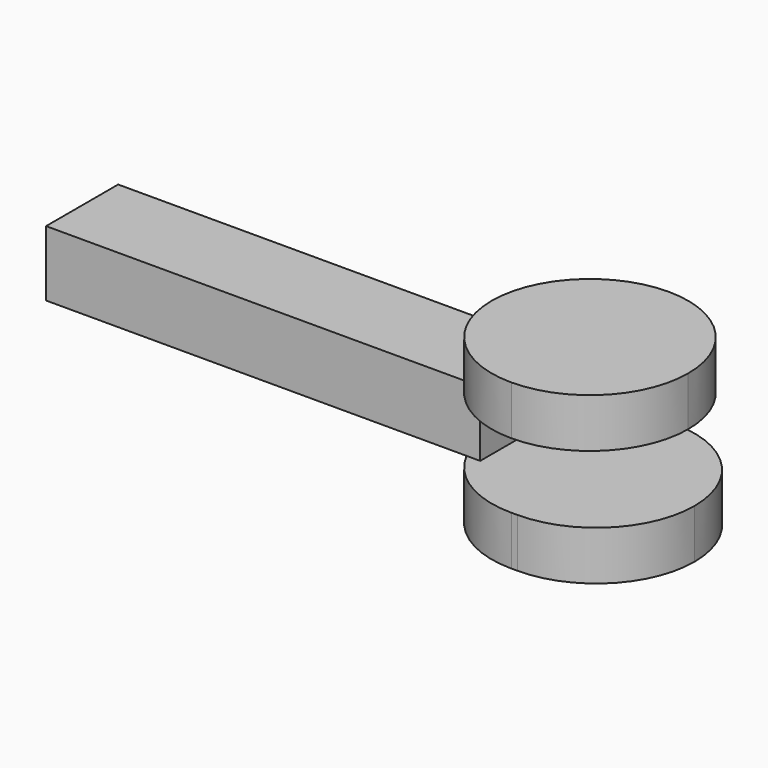
from build123d import *

# Parameters (mm, degrees)
F1_DEPTH = 24
F2_DEPTH = 11
F3_R     = 23.99999
F3_2_R   = 23.99999


# Not quite as in the source:
# - a fillet or chamfer is up to 0.001 mm smaller than in the source, because OpenCascade refuses the exact size


with BuildPart() as f1:
    # F0 (on Front) → F1 (new body, symmetric)
    with BuildSketch(Plane.XZ):
        Polygon((28.0138015747, 20.5115029328), (28.0138015747, 8.5115029328), (34.0138015747, 8.5115029328), (76.0138015747, 8.5115029328), (76.0138015747, 20.5115029328), align=None)
    extrude(amount=F1_DEPTH, both=True)

    # F3 (radius 24 in the source; OpenCascade refuses exactly that, so slightly less here)
    f3_edges = [f1.edges().sort_by_distance(p)[0] for p in [
        (76.013802, -24, 14.511503),
        (76.013802, 24, 14.511503),
        (28.013802, -24, 14.511503),
        (28.013802, 24, 14.511503),
    ]]
    fillet(f3_edges, radius=F3_R)


with BuildPart() as f1b:
    # F0 (on Front) → F1, piece 2 (new body, symmetric)
    with BuildSketch(Plane.XZ):
        Polygon((34.0138015747, -7.4884970672), (28.0138015747, -7.4884970672), (28.0138015747, -19.4884970672), (77.5421783328, -19.4884970672), (77.5421783328, -7.4884970672), align=None)
    extrude(amount=F1_DEPTH, both=True)

    # F3#2 (radius 24 in the source; OpenCascade refuses exactly that, so slightly less here)
    f3_2_edges = [f1b.edges().sort_by_distance(p)[0] for p in [
        (77.542178, 24, -13.488497),
        (77.542178, -24, -13.488497),
        (28.013802, -24, -13.488497),
        (28.013802, 24, -13.488497),
    ]]
    fillet(f3_2_edges, radius=F3_2_R)


with BuildPart() as f2:
    # F0 (on Front) → F2 (new body, symmetric)
    with BuildSketch(Plane.XZ):
        Polygon((28.0138015747, 8.5115029328), (-71.9861984253, 8.5115029328), (-71.9861984253, -7.4884970672), (28.0138015747, -7.4884970672), (34.0138015747, -7.4884970672), (34.0138015747, 8.5115029328), align=None)
    extrude(amount=F2_DEPTH, both=True)


solid = Compound([f1.part, f1b.part, f2.part])
